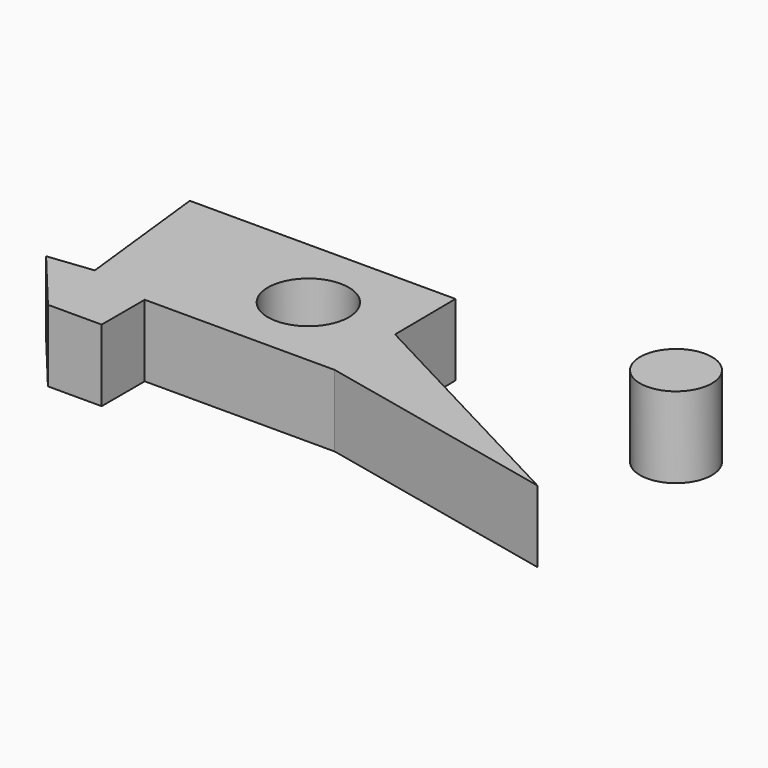
from build123d import *

# Parameters (mm, degrees)
F0_R     = 2.25
F1_DEPTH = 4
F0_R_2   = 2
F2_DEPTH = 4.5


# Not quite as in the source:
# - a feature names something its author has since deleted; it is built from what else it names


with BuildPart() as f1:
    # F0 (on Top) → F1 (new body)
    with BuildSketch(Plane.XY):
        Polygon((-8.6991069838, -7.25), (-5.7089743204, -7.25), (-5.7089743204, -4.25), (4.8668961972, -4.25), (4.8295045272, 0), (4.7921128571, 4.25), (-10, 4.25), (-9.1290873029, -3.4489390308), align=None)
        Circle(F0_R, mode=Mode.SUBTRACT)
        Polygon((4.8295045272, 0), (4.8668961972, -4.25), (18.5611117631, -7.25), align=None)
        Polygon((-11.6174062714, -3.7304204889), (-8.6991069838, -7.25), (-9.1290873029, -3.4489390308), align=None)
    extrude(amount=F1_DEPTH)


with BuildPart() as f2:
    # F0 (on Top) → F2 (new body)
    with BuildSketch(Plane.XY):
        with Locations((17.0693118125, 4.25)):
            Circle(F0_R_2)
    extrude(amount=F2_DEPTH)


solid = Compound([f1.part, f2.part])
